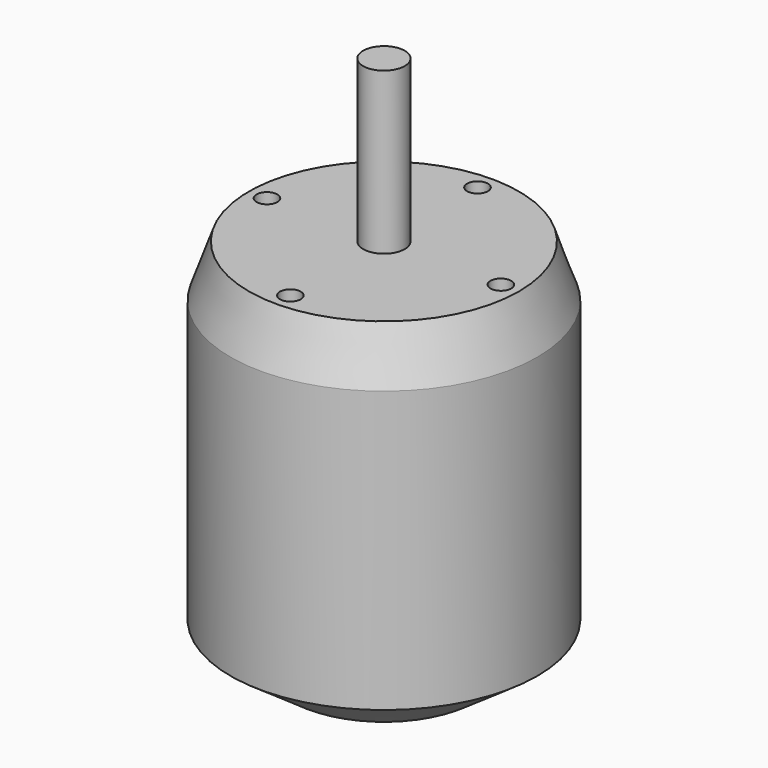
from build123d import *

# Parameters (mm, degrees)
F0_R     = 29.5
F1_DEPTH = 72
F3_SIZE2 = 11.5
F3_SIZE  = 8
F4_R     = 4
F5_DEPTH = 103
F7_D     = 4
F7_DEPTH = 20
F7_TIP   = 1.2017212381


# Not quite as in the source:
# - a fillet or chamfer that OpenCascade refuses, or shapes differently, is made with other operations: its cross-section is extruded or revolved along the edge and cut away or added


with BuildPart() as f1:
    # F0 (on Top) → F1 (new body)
    with BuildSketch(Plane.XY):
        Circle(F0_R)
    extrude(amount=F1_DEPTH)

    # F2: chamfer of 3.5 x 10 on 1 edges, made by hand

    # F2_s1 → F2_t2 (revolve, cut)
    with BuildSketch(Plane.XZ):
        Polygon((29.5, 62), (26, 72), (29.5, 72), align=None)
    revolve(axis=Axis((0, 0, 72), (0, 0, 1)), mode=Mode.SUBTRACT)

    # F3
    f3_edges = [f1.edges().sort_by_distance(p)[0] for p in [
        (-29.5, 0, 0),
    ]]
    chamfer(f3_edges, length=F3_SIZE, length2=F3_SIZE2)

    # F4 (on Top) → F5 (join)
    with BuildSketch(Plane.XY):
        Circle(F4_R)
    extrude(amount=F5_DEPTH)

    # F7
    with Locations(Plane.XY.offset(72)):
        with Locations((0, 22.5), (22.5, 0), (0, -22.5), (-22.5, 0)):
            Hole(F7_D / 2, depth=F7_DEPTH)
            with Locations((0, 0, -(F7_DEPTH + F7_TIP / 2))):  # 118° drill point
                Cone(0, F7_D / 2, F7_TIP, mode=Mode.SUBTRACT)


solid = f1.part
